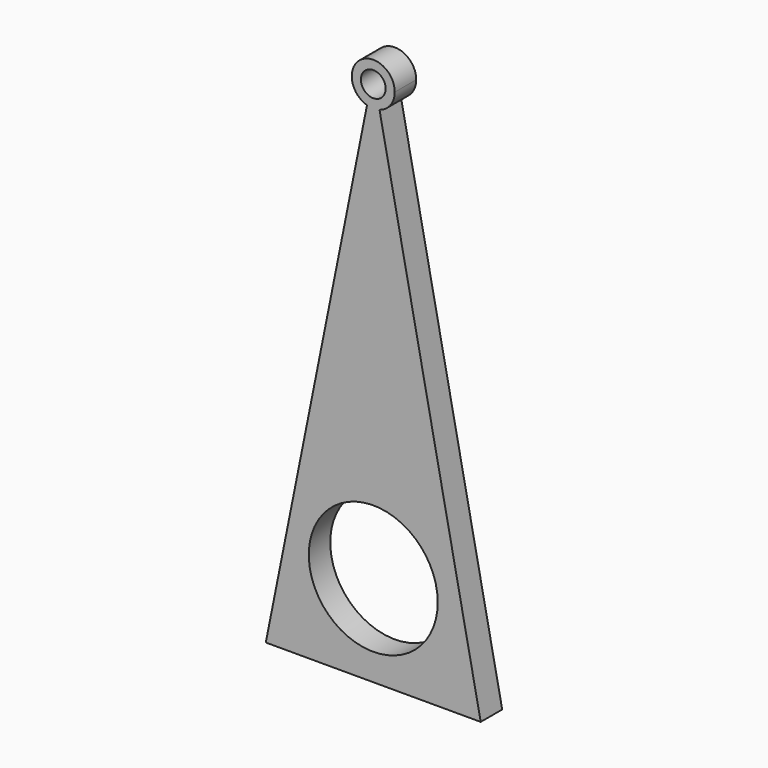
from build123d import *

# Parameters (mm, degrees)
F1_DEPTH = 3.175
F2_R     = 7.62
F3_DEPTH = 3.176
F5_DEPTH = 3.175
F6_R     = 1.4652480926
F7_DEPTH = 3.176


with BuildPart() as f1:
    # F0 (on Front) → F1 (new body)
    with BuildSketch(Plane.XZ):
        Polygon((12.7, -25.4), (0, 38.1), (-12.7, -25.4), align=None)
    extrude(amount=F1_DEPTH)

    # F2 (on face) → F3 (cut, through all)
    with BuildSketch(Plane.XZ.offset(3.175)):
        with Locations((0, -14.6123587166)):
            Circle(F2_R)
    extrude(amount=-F3_DEPTH, mode=Mode.SUBTRACT)

    # F4 (on face) → F5 (join, through all)
    with BuildSketch(Plane.XZ.offset(3.175)):
        with BuildLine():
            ThreePointArc((0.739965088, 34.4001745601), (2.0409692947, 35.3180329573), (2.54, 36.83))
            ThreePointArc((2.54, 36.83), (-1.5119670427, 38.8709692947), (-0.739965088, 34.4001745601))
            Line((-0.739965088, 34.4001745601), (0, 38.1))
            Line((0, 38.1), (0.739965088, 34.4001745601))
        make_face()
    extrude(amount=-F5_DEPTH)

    # F6 (on face) → F7 (cut, through all)
    with BuildSketch(Plane.XZ.offset(3.175)):
        with Locations((0, 36.83)):
            Circle(F6_R)
    extrude(amount=-F7_DEPTH, mode=Mode.SUBTRACT)


solid = f1.part
